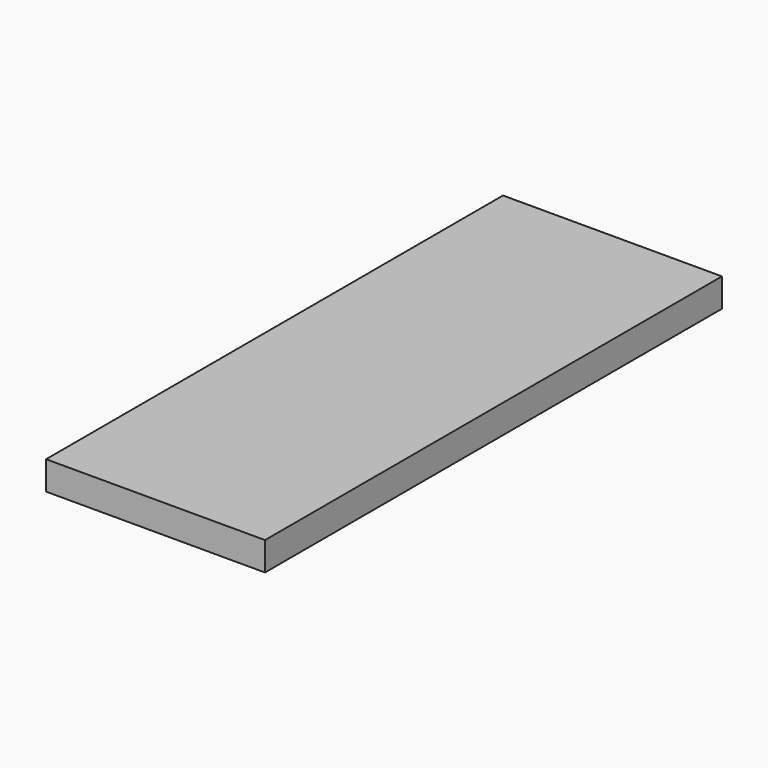
from build123d import *

# Parameters (mm, degrees)
F0_W     = 146.05
F0_H     = 381
F1_DEPTH = 19.05


# Not quite as in the source:
# - a length typed as a fraction of an inch, garbled in the dataset ("3 / 203.2 mm" for 3/8 in), is restored


with BuildPart() as f1:
    # F0 (on Top) → F1 (new body)
    with BuildSketch(Plane.XY):
        with Locations((0.6443743676, 117.0459133416)):
            Rectangle(F0_W, F0_H)
    extrude(amount=F1_DEPTH)


solid = f1.part
